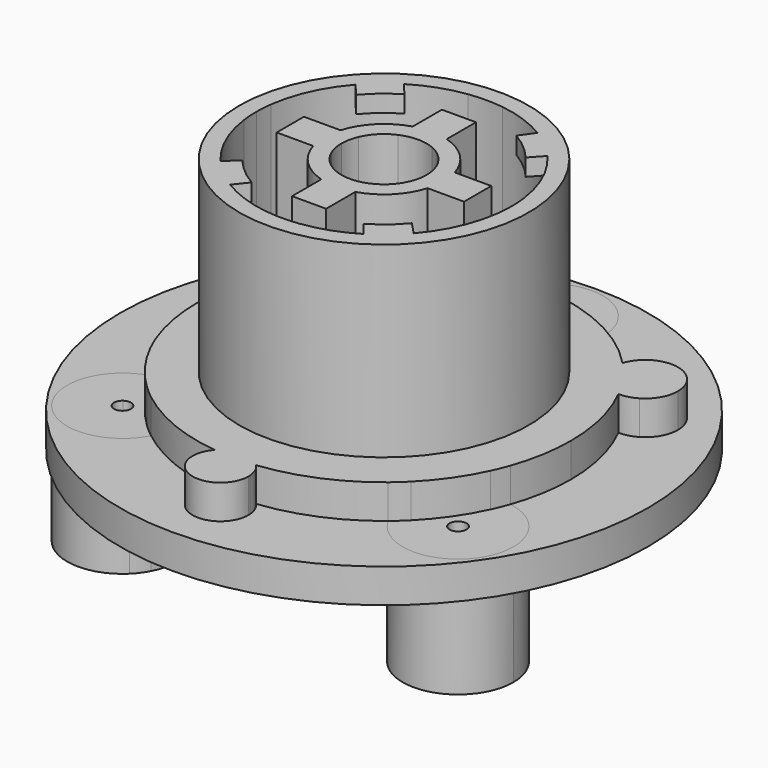
from build123d import *
from build123d import SkipClean  # not in build123d's __all__

# Parameters (mm, degrees)
F1_DEPTH  = 2
F2_DEPTH  = 15
F3_DEPTH  = 5
F4_DEPTH  = 4
F5_DEPTH  = 2
F6_DEPTH  = 1
F7_DEPTH  = 2
F8_DEPTH  = 14.99
F9_DEPTH  = 4
F12_DEPTH = 1
F14_R     = 7.5
F14_R_2   = 2.5
F15_DEPTH = 2
F16_DEPTH = 20.001


# Not quite as in the source:
# - a feature names something its author has since deleted; it is built from what else it names


with BuildPart() as f1:
    # F0 (on Top) → F1 (new body)
    with BuildSketch(Plane.XY):
        with BuildLine():
            Line((12, 0), (15.5, 0))
            ThreePointArc((15.5, 0), (0, 15.5), (-15.5, 0))
            Line((-15.5, 0), (-12, 0))
            ThreePointArc((-12, 0), (-11.6801289605, 2.7521968435), (-10.7375687557, 5.3576690095))
            ThreePointArc((-10.7375687557, 5.3576690095), (-11.2889375611, 7.9513228909), (-8.6611158458, 8.3057252727))
            ThreePointArc((-8.6611158458, 8.3057252727), (-6.1593840275, 10.2986401239), (-3.2200634035, 11.5598958333))
            ThreePointArc((-3.2200634035, 11.5598958333), (-0.2205605797, 15.2425072137), (3.25, 12))
            ThreePointArc((3.25, 12), (3.2425072137, 11.7794394203), (3.2200634035, 11.5598958333))
            ThreePointArc((3.2200634035, 11.5598958333), (6.111431372, 10.3271683721), (8.5835031281, 8.385909256))
            ThreePointArc((8.5835031281, 8.385909256), (10.6257203534, 8.6478632276), (11.7300664525, 6.9101374805))
            ThreePointArc((11.7300664525, 6.9101374805), (11.4776891115, 5.9587644605), (10.786927533, 5.2575844642))
            ThreePointArc((10.786927533, 5.2575844642), (11.692799716, 2.6978574466), (12, 0))
        make_face()
        with BuildLine():
            ThreePointArc((-15.5, 0), (0, -15.5), (15.5, 0))
            Line((15.5, 0), (12, 0))
            ThreePointArc((12, 0), (11.8294726454, -2.0158315735), (11.3227371779, -3.9743707428))
            ThreePointArc((11.3227371779, -3.9743707428), (12.6139140233, -5.1718208797), (13.090994712, -6.8669369503))
            ThreePointArc((13.090994712, -6.8669369503), (11.1449971369, -9.8438611475), (7.6374084499, -9.2558085638))
            ThreePointArc((7.6374084499, -9.2558085638), (4.8184795385, -10.9900980404), (1.6330075435, -11.8883676913))
            ThreePointArc((1.6330075435, -11.8883676913), (1.6358656226, -11.9441513269), (1.6368186856, -12))
            ThreePointArc((1.6368186856, -12), (-0.0558486731, -13.6358656226), (-1.6330075435, -11.8883676913))
            ThreePointArc((-1.6330075435, -11.8883676913), (-4.6750940722, -11.0518548405), (-7.3940132882, -9.4513791319))
            ThreePointArc((-7.3940132882, -9.4513791319), (-12.2749858869, -9.0491558433), (-11.2155025424, -4.2676108915))
            ThreePointArc((-11.2155025424, -4.2676108915), (-11.8022461953, -2.1695586523), (-12, 0))
            Line((-12, 0), (-15.5, 0))
        make_face()
        with BuildLine():
            Line((8.5, 0), (10.9707452996, 0))
            ThreePointArc((10.9707452996, 0), (10.6662314199, 2.5668579481), (9.7695945034, 4.9912198577))
            ThreePointArc((9.7695945034, 4.9912198577), (8.2415199443, 5.804885166), (7.9900576645, 7.5177277782))
            ThreePointArc((7.9900576645, 7.5177277782), (5.6655330905, 9.3946254438), (2.92083067, 10.5747813512))
            ThreePointArc((2.92083067, 10.5747813512), (0, 8.75), (-2.92083067, 10.5747813512))
            ThreePointArc((-2.92083067, 10.5747813512), (-5.7202127626, 9.3614324961), (-8.0771781233, 7.4240451232))
            ThreePointArc((-8.0771781233, 7.4240451232), (-8.0213473893, 7.1697823433), (-8.0026076616, 6.9101374805))
            ThreePointArc((-8.0026076616, 6.9101374805), (-8.4973152844, 5.667468241), (-9.7107279849, 5.1048030747))
            ThreePointArc((-9.7107279849, 5.1048030747), (-10.6510838844, 2.6290044725), (-10.9707452996, 0))
            Line((-10.9707452996, 0), (-8.5, 0))
            ThreePointArc((-8.5, 0), (0, 8.5), (8.5, 0))
        make_face()
        with BuildLine():
            ThreePointArc((10.3436272842, -3.6560398019), (10.8128292513, -1.8547172317), (10.9707452996, 0))
            Line((10.9707452996, 0), (8.5, 0))
            ThreePointArc((8.5, 0), (0, -8.5), (-8.5, 0))
            Line((-8.5, 0), (-10.9707452996, 0))
            ThreePointArc((-10.9707452996, 0), (-10.7877848856, -1.9952317382), (-10.2450061487, -3.9239140461))
            ThreePointArc((-10.2450061487, -3.9239140461), (-7.578380718, -4.6239491218), (-6.409005288, -7.120647221))
            ThreePointArc((-6.409005288, -7.120647221), (-6.5027661125, -7.8956661027), (-6.7786386831, -8.625967194))
            ThreePointArc((-6.7786386831, -8.625967194), (-4.1558671902, -10.1531285979), (-1.2150398702, -10.9032532091))
            ThreePointArc((-1.2150398702, -10.9032532091), (0, -10.3631813144), (1.2150398702, -10.9032532091))
            ThreePointArc((1.2150398702, -10.9032532091), (4.2876044557, -10.0982028331), (7.0007672753, -8.4466863317))
            ThreePointArc((7.0007672753, -8.4466863317), (7.1757253108, -5.0071415263), (10.3436272842, -3.6560398019))
        make_face()
        with BuildLine():
            ThreePointArc((-6.7786386831, -8.625967194), (-7.053433372, -9.0631958021), (-7.3940132882, -9.4513791319))
            ThreePointArc((-7.3940132882, -9.4513791319), (-4.6750940722, -11.0518548405), (-1.6330075435, -11.8883676913))
            ThreePointArc((-1.6330075435, -11.8883676913), (-1.5068032896, -11.3606884515), (-1.2150398702, -10.9032532091))
            ThreePointArc((-1.2150398702, -10.9032532091), (-4.1558671902, -10.1531285979), (-6.7786386831, -8.625967194))
        make_face()
        with BuildLine():
            Line((-10.9707452996, 0), (-12, 0))
            ThreePointArc((-12, 0), (-11.8022461953, -2.1695586523), (-11.2155025424, -4.2676108915))
            ThreePointArc((-11.2155025424, -4.2676108915), (-10.7439506432, -4.0570882487), (-10.2450061487, -3.9239140461))
            ThreePointArc((-10.2450061487, -3.9239140461), (-10.7877848856, -1.9952317382), (-10.9707452996, 0))
        make_face()
        with BuildLine():
            ThreePointArc((-10.7375687557, 5.3576690095), (-11.6801289605, 2.7521968435), (-12, 0))
            Line((-12, 0), (-10.9707452996, 0))
            ThreePointArc((-10.9707452996, 0), (-10.6510838844, 2.6290044725), (-9.7107279849, 5.1048030747))
            ThreePointArc((-9.7107279849, 5.1048030747), (-10.2430484347, 5.1544864526), (-10.7375687557, 5.3576690095))
        make_face()
        with BuildLine():
            ThreePointArc((-3.2200634035, 11.5598958333), (-6.1593840275, 10.2986401239), (-8.6611158458, 8.3057252727))
            ThreePointArc((-8.6611158458, 8.3057252727), (-8.3032471961, 7.9085306996), (-8.0771781233, 7.4240451232))
            ThreePointArc((-8.0771781233, 7.4240451232), (-5.7202127626, 9.3614324961), (-2.92083067, 10.5747813512))
            ThreePointArc((-2.92083067, 10.5747813512), (-3.1097037867, 11.0554141867), (-3.2200634035, 11.5598958333))
        make_face()
        with BuildLine():
            ThreePointArc((2.92083067, 10.5747813512), (5.6655330905, 9.3946254438), (7.9900576645, 7.5177277782))
            ThreePointArc((7.9900576645, 7.5177277782), (8.2261607277, 7.9932550925), (8.5835031281, 8.385909256))
            ThreePointArc((8.5835031281, 8.385909256), (6.111431372, 10.3271683721), (3.2200634035, 11.5598958333))
            ThreePointArc((3.2200634035, 11.5598958333), (3.1097037867, 11.0554141867), (2.92083067, 10.5747813512))
        make_face()
        with BuildLine():
            Line((10.9707452996, 0), (12, 0))
            ThreePointArc((12, 0), (11.692799716, 2.6978574466), (10.786927533, 5.2575844642))
            ThreePointArc((10.786927533, 5.2575844642), (10.2968595884, 5.0533681748), (9.7695945034, 4.9912198577))
            ThreePointArc((9.7695945034, 4.9912198577), (10.6662314199, 2.5668579481), (10.9707452996, 0))
        make_face()
        with BuildLine():
            ThreePointArc((11.3227371779, -3.9743707428), (11.8294726454, -2.0158315735), (12, 0))
            Line((12, 0), (10.9707452996, 0))
            ThreePointArc((10.9707452996, 0), (10.8128292513, -1.8547172317), (10.3436272842, -3.6560398019))
            ThreePointArc((10.3436272842, -3.6560398019), (10.8458676989, -3.7761878049), (11.3227371779, -3.9743707428))
        make_face()
        with BuildLine():
            ThreePointArc((7.6374084499, -9.2558085638), (7.2868443927, -8.8766175584), (7.0007672753, -8.4466863317))
            ThreePointArc((7.0007672753, -8.4466863317), (4.2876044557, -10.0982028331), (1.2150398702, -10.9032532091))
            ThreePointArc((1.2150398702, -10.9032532091), (1.5068032896, -11.3606884515), (1.6330075435, -11.8883676913))
            ThreePointArc((1.6330075435, -11.8883676913), (4.8184795385, -10.9900980404), (7.6374084499, -9.2558085638))
        make_face()
    extrude(amount=F1_DEPTH)

    # F0 (on Top) → F2 (join)
    with BuildSketch(Plane.XY):
        with BuildLine():
            Line((7.5, 0), (8.5, 0))
            ThreePointArc((8.5, 0), (0, 8.5), (-8.5, 0))
            Line((-8.5, 0), (-7.5, 0))
            ThreePointArc((-7.5, 0), (-7.4832398666, 0.5011198447), (-7.4330343737, 1))
            ThreePointArc((-7.4330343737, 1), (-5.3033008589, 5.3033008589), (-1, 7.4330343737))
            ThreePointArc((-1, 7.4330343737), (0, 7.5), (1, 7.4330343737))
            ThreePointArc((1, 7.4330343737), (5.3033008589, 5.3033008589), (7.4330343737, 1))
            ThreePointArc((7.4330343737, 1), (7.4832398666, 0.5011198447), (7.5, 0))
        make_face()
        with BuildLine():
            ThreePointArc((-8.5, 0), (0, -8.5), (8.5, 0))
            Line((8.5, 0), (7.5, 0))
            ThreePointArc((7.5, 0), (7.4832398666, -0.5011198447), (7.4330343737, -1))
            ThreePointArc((7.4330343737, -1), (5.3033008589, -5.3033008589), (1, -7.4330343737))
            ThreePointArc((1, -7.4330343737), (0, -7.5), (-1, -7.4330343737))
            ThreePointArc((-1, -7.4330343737), (-5.3033008589, -5.3033008589), (-7.4330343737, -1))
            ThreePointArc((-7.4330343737, -1), (-7.4832398666, -0.5011198447), (-7.5, 0))
            Line((-7.5, 0), (-8.5, 0))
        make_face()
    extrude(amount=F2_DEPTH)

    # F11 (on offset) → F12 (join)
    with BuildSketch(Plane.XY.offset(15)):
        with BuildLine():
            ThreePointArc((3.9228129696, -6.3923030596), (4.8521590221, -5.718964314), (5.6678938929, -4.9117185199))
            Line((5.6678938929, -4.9117185199), (4.9799266597, -4.1773592692))
            ThreePointArc((4.9799266597, -4.1773592692), (4.1945547803, -4.9654516607), (3.2862850661, -5.6080594205))
            Line((3.2862850661, -5.6080594205), (3.9228129696, -6.3923030596))
        make_face()
        with BuildLine():
            ThreePointArc((-5.7358275815, -4.832212946), (-4.890446416, -5.686258335), (-3.9195165937, -6.3943248018))
            Line((-3.9195165937, -6.3943248018), (-3.2862850661, -5.6080594205))
            ThreePointArc((-3.2862850661, -5.6080594205), (-4.1945547803, -4.9654516607), (-4.9799266597, -4.1773592692))
            Line((-4.9799266597, -4.1773592692), (-5.7358275815, -4.832212946))
        make_face()
        with BuildLine():
            Line((4.9799266597, 4.1773592692), (5.6618978404, 4.9186291632))
            ThreePointArc((5.6618978404, 4.9186291632), (4.8270188563, 5.7401993834), (3.8744034722, 6.421759707))
            Line((3.8744034722, 6.421759707), (3.2862850661, 5.6080594205))
            ThreePointArc((3.2862850661, 5.6080594205), (4.1945547803, 4.9654516607), (4.9799266597, 4.1773592692))
        make_face()
        with BuildLine():
            Line((-3.2862850661, 5.6080594205), (-3.9398925434, 6.3817902462))
            ThreePointArc((-3.9398925434, 6.3817902462), (-4.8398709003, 5.7293673009), (-5.633534137, 4.9510900949))
            Line((-5.633534137, 4.9510900949), (-4.9799266597, 4.1773592692))
            ThreePointArc((-4.9799266597, 4.1773592692), (-4.1945547803, 4.9654516607), (-3.2862850661, 5.6080594205))
        make_face()
    extrude(amount=-F12_DEPTH)


with BuildPart() as f3:
    # F0 (on Top) → F3 (new body)
    with BuildSketch(Plane.XY):
        with BuildLine():
            ThreePointArc((3.25, 12), (-0.2205605797, 15.2425072137), (-3.2200634035, 11.5598958333))
            ThreePointArc((-3.2200634035, 11.5598958333), (-2.7324804918, 11.6847571803), (-2.2400905501, 11.7890624872))
            ThreePointArc((-2.2400905501, 11.7890624872), (-0.1055850757, 14.2475213234), (2.2500000683, 12))
            ThreePointArc((2.2500000683, 12), (2.2475213234, 11.8944149243), (2.2400905501, 11.7890624872))
            ThreePointArc((2.2400905501, 11.7890624872), (2.7324804918, 11.6847571803), (3.2200634035, 11.5598958333))
            ThreePointArc((3.2200634035, 11.5598958333), (3.2425072137, 11.7794394203), (3.25, 12))
        make_face()
        with BuildLine():
            ThreePointArc((1.9057701678, 10.803948005), (2.4160190916, 10.7014066448), (2.92083067, 10.5747813512))
            ThreePointArc((2.92083067, 10.5747813512), (3.1097037867, 11.0554141867), (3.2200634035, 11.5598958333))
            ThreePointArc((3.2200634035, 11.5598958333), (2.7324804918, 11.6847571803), (2.2400905501, 11.7890624872))
            ThreePointArc((2.2400905501, 11.7890624872), (2.1306461248, 11.2769181248), (1.9057701678, 10.803948005))
        make_face()
        with BuildLine():
            ThreePointArc((-2.92083067, 10.5747813512), (0, 8.75), (2.92083067, 10.5747813512))
            ThreePointArc((2.92083067, 10.5747813512), (2.4160190916, 10.7014066448), (1.9057701678, 10.803948005))
            ThreePointArc((1.9057701678, 10.803948005), (0, 9.7499999317), (-1.9057701678, 10.803948005))
            ThreePointArc((-1.9057701678, 10.803948005), (-2.4160190916, 10.7014066448), (-2.92083067, 10.5747813512))
        make_face()
        with BuildLine():
            ThreePointArc((-2.2400905501, 11.7890624872), (-2.7324804918, 11.6847571803), (-3.2200634035, 11.5598958333))
            ThreePointArc((-3.2200634035, 11.5598958333), (-3.1097037867, 11.0554141867), (-2.92083067, 10.5747813512))
            ThreePointArc((-2.92083067, 10.5747813512), (-2.4160190916, 10.7014066448), (-1.9057701678, 10.803948005))
            ThreePointArc((-1.9057701678, 10.803948005), (-2.1306461248, 11.2769181248), (-2.2400905501, 11.7890624872))
        make_face()
    extrude(amount=-F3_DEPTH)


with BuildPart() as f3b:
    # F0 (on Top) → F3, piece 2 (new body)
    with BuildSketch(Plane.XY):
        with BuildLine():
            ThreePointArc((7.7695659726, -7.7453919865), (7.3934862888, -8.1051596483), (7.0007672753, -8.4466863317))
            ThreePointArc((7.0007672753, -8.4466863317), (7.2868443927, -8.8766175584), (7.6374084499, -9.2558085638))
            ThreePointArc((7.6374084499, -9.2558085638), (8.0188218667, -8.9274014063), (8.3861284242, -8.5832889997))
            ThreePointArc((8.3861284242, -8.5832889997), (8.0287565914, -8.2004635781), (7.7695659726, -7.7453919865))
        make_face()
        with BuildLine():
            ThreePointArc((13.090994712, -6.8669369503), (12.6139140233, -5.1718208797), (11.3227371779, -3.9743707428))
            ThreePointArc((11.3227371779, -3.9743707428), (11.1461170716, -4.4456804007), (10.9498885107, -4.9091691357))
            ThreePointArc((10.9498885107, -4.9091691357), (11.784896894, -5.7339124231), (12.0909947725, -6.8669369503))
            ThreePointArc((12.0909947725, -6.8669369503), (10.7867883039, -8.9084987921), (8.3861284242, -8.5832889997))
            ThreePointArc((8.3861284242, -8.5832889997), (8.0188218667, -8.9274014063), (7.6374084499, -9.2558085638))
            ThreePointArc((7.6374084499, -9.2558085638), (11.1449971369, -9.8438611475), (13.090994712, -6.8669369503))
        make_face()
        with BuildLine():
            ThreePointArc((9.950699894, -4.619612976), (10.1585947463, -4.1424878043), (10.3436272842, -3.6560398019))
            ThreePointArc((10.3436272842, -3.6560398019), (7.1757253108, -5.0071415263), (7.0007672753, -8.4466863317))
            ThreePointArc((7.0007672753, -8.4466863317), (7.3934862888, -8.1051596483), (7.7695659726, -7.7453919865))
            ThreePointArc((7.7695659726, -7.7453919865), (7.9958081538, -5.5793862374), (9.950699894, -4.619612976))
        make_face()
        with BuildLine():
            ThreePointArc((10.9498885107, -4.9091691357), (11.1461170716, -4.4456804007), (11.3227371779, -3.9743707428))
            ThreePointArc((11.3227371779, -3.9743707428), (10.8458676989, -3.7761878049), (10.3436272842, -3.6560398019))
            ThreePointArc((10.3436272842, -3.6560398019), (10.1585947463, -4.1424878043), (9.950699894, -4.619612976))
            ThreePointArc((9.950699894, -4.619612976), (10.467258683, -4.7058507162), (10.9498885107, -4.9091691357))
        make_face()
    extrude(amount=-F3_DEPTH)


with BuildPart() as f3c:
    # F0 (on Top) → F3, piece 3 (new body)
    with BuildSketch(Plane.XY):
        with BuildLine():
            ThreePointArc((-10.818459234, -5.1923924931), (-11.0266800599, -4.7341659092), (-11.2155025424, -4.2676108915))
            ThreePointArc((-11.2155025424, -4.2676108915), (-12.2749858869, -9.0491558433), (-7.3940132882, -9.4513791319))
            ThreePointArc((-7.3940132882, -9.4513791319), (-7.7838418619, -9.1330063982), (-8.1599769543, -8.7985667074))
            ThreePointArc((-8.1599769543, -8.7985667074), (-11.4700687346, -8.4557685417), (-10.818459234, -5.1923924931))
        make_face()
        with BuildLine():
            ThreePointArc((-10.2450061487, -3.9239140461), (-10.7439506432, -4.0570882487), (-11.2155025424, -4.2676108915))
            ThreePointArc((-11.2155025424, -4.2676108915), (-11.0266800599, -4.7341659092), (-10.818459234, -5.1923924931))
            ThreePointArc((-10.818459234, -5.1923924931), (-10.3412825445, -4.9765862391), (-9.8271422706, -4.8769383041))
            ThreePointArc((-9.8271422706, -4.8769383041), (-10.0473802232, -4.4053834201), (-10.2450061487, -3.9239140461))
        make_face()
        with BuildLine():
            ThreePointArc((-6.409005288, -7.120647221), (-7.578380718, -4.6239491218), (-10.2450061487, -3.9239140461))
            ThreePointArc((-10.2450061487, -3.9239140461), (-10.0473802232, -4.4053834201), (-9.8271422706, -4.8769383041))
            ThreePointArc((-9.8271422706, -4.8769383041), (-8.1286145623, -5.4712825024), (-7.4090053439, -7.120647221))
            ThreePointArc((-7.4090053439, -7.120647221), (-7.448455587, -7.5401347268), (-7.565422919, -7.9449121131))
            ThreePointArc((-7.565422919, -7.9449121131), (-7.1801103625, -8.2947735117), (-6.7786386831, -8.625967194))
            ThreePointArc((-6.7786386831, -8.625967194), (-6.5027661125, -7.8956661027), (-6.409005288, -7.120647221))
        make_face()
        with BuildLine():
            ThreePointArc((-8.1599769543, -8.7985667074), (-7.7838418619, -9.1330063982), (-7.3940132882, -9.4513791319))
            ThreePointArc((-7.3940132882, -9.4513791319), (-7.053433372, -9.0631958021), (-6.7786386831, -8.625967194))
            ThreePointArc((-6.7786386831, -8.625967194), (-7.1801103625, -8.2947735117), (-7.565422919, -7.9449121131))
            ThreePointArc((-7.565422919, -7.9449121131), (-7.8126861236, -8.4065730708), (-8.1599769543, -8.7985667074))
        make_face()
    extrude(amount=-F3_DEPTH)


with BuildPart() as f4:
    # F0 (on Top) → F4 (new body)
    with BuildSketch(Plane.XY):
        with BuildLine():
            ThreePointArc((10.3436272842, -3.6560398019), (10.8128292513, -1.8547172317), (10.9707452996, 0))
            Line((10.9707452996, 0), (8.5, 0))
            ThreePointArc((8.5, 0), (0, -8.5), (-8.5, 0))
            Line((-8.5, 0), (-10.9707452996, 0))
            ThreePointArc((-10.9707452996, 0), (-10.7877848856, -1.9952317382), (-10.2450061487, -3.9239140461))
            ThreePointArc((-10.2450061487, -3.9239140461), (-7.578380718, -4.6239491218), (-6.409005288, -7.120647221))
            ThreePointArc((-6.409005288, -7.120647221), (-6.5027661125, -7.8956661027), (-6.7786386831, -8.625967194))
            ThreePointArc((-6.7786386831, -8.625967194), (-4.1558671902, -10.1531285979), (-1.2150398702, -10.9032532091))
            ThreePointArc((-1.2150398702, -10.9032532091), (0, -10.3631813144), (1.2150398702, -10.9032532091))
            ThreePointArc((1.2150398702, -10.9032532091), (4.2876044557, -10.0982028331), (7.0007672753, -8.4466863317))
            ThreePointArc((7.0007672753, -8.4466863317), (7.1757253108, -5.0071415263), (10.3436272842, -3.6560398019))
        make_face()
        with BuildLine():
            Line((8.5, 0), (10.9707452996, 0))
            ThreePointArc((10.9707452996, 0), (10.6662314199, 2.5668579481), (9.7695945034, 4.9912198577))
            ThreePointArc((9.7695945034, 4.9912198577), (8.2415199443, 5.804885166), (7.9900576645, 7.5177277782))
            ThreePointArc((7.9900576645, 7.5177277782), (5.6655330905, 9.3946254438), (2.92083067, 10.5747813512))
            ThreePointArc((2.92083067, 10.5747813512), (0, 8.75), (-2.92083067, 10.5747813512))
            ThreePointArc((-2.92083067, 10.5747813512), (-5.7202127626, 9.3614324961), (-8.0771781233, 7.4240451232))
            ThreePointArc((-8.0771781233, 7.4240451232), (-8.0213473893, 7.1697823433), (-8.0026076616, 6.9101374805))
            ThreePointArc((-8.0026076616, 6.9101374805), (-8.4973152844, 5.667468241), (-9.7107279849, 5.1048030747))
            ThreePointArc((-9.7107279849, 5.1048030747), (-10.6510838844, 2.6290044725), (-10.9707452996, 0))
            Line((-10.9707452996, 0), (-8.5, 0))
            ThreePointArc((-8.5, 0), (0, 8.5), (8.5, 0))
        make_face()
        with BuildLine():
            ThreePointArc((-6.409005288, -7.120647221), (-7.578380718, -4.6239491218), (-10.2450061487, -3.9239140461))
            ThreePointArc((-10.2450061487, -3.9239140461), (-10.0473802232, -4.4053834201), (-9.8271422706, -4.8769383041))
            ThreePointArc((-9.8271422706, -4.8769383041), (-8.1286145623, -5.4712825024), (-7.4090053439, -7.120647221))
            ThreePointArc((-7.4090053439, -7.120647221), (-7.448455587, -7.5401347268), (-7.565422919, -7.9449121131))
            ThreePointArc((-7.565422919, -7.9449121131), (-7.1801103625, -8.2947735117), (-6.7786386831, -8.625967194))
            ThreePointArc((-6.7786386831, -8.625967194), (-6.5027661125, -7.8956661027), (-6.409005288, -7.120647221))
        make_face()
        with BuildLine():
            ThreePointArc((-7.4090053439, -7.120647221), (-8.1286145623, -5.4712825024), (-9.8271422706, -4.8769383041))
            ThreePointArc((-9.8271422706, -4.8769383041), (-8.8305405719, -6.5099005858), (-7.565422919, -7.9449121131))
            ThreePointArc((-7.565422919, -7.9449121131), (-7.448455587, -7.5401347268), (-7.4090053439, -7.120647221))
        make_face()
        with BuildLine():
            ThreePointArc((-8.0771781233, 7.4240451232), (-8.9692319542, 6.3174465237), (-9.7107279849, 5.1048030747))
            ThreePointArc((-9.7107279849, 5.1048030747), (-8.4973152844, 5.667468241), (-8.0026076616, 6.9101374805))
            ThreePointArc((-8.0026076616, 6.9101374805), (-8.0213473893, 7.1697823433), (-8.0771781233, 7.4240451232))
        make_face()
        with BuildLine():
            ThreePointArc((-8.6611158458, 8.3057252727), (-11.2889375611, 7.9513228909), (-10.7375687557, 5.3576690095))
            ThreePointArc((-10.7375687557, 5.3576690095), (-10.5507798679, 5.7167336984), (-10.351988183, 6.0692949063))
            ThreePointArc((-10.351988183, 6.0692949063), (-10.6282674714, 7.4859822706), (-9.2012987677, 7.7029929889))
            ThreePointArc((-9.2012987677, 7.7029929889), (-8.9362903661, 8.0089146888), (-8.6611158458, 8.3057252727))
        make_face()
        with BuildLine():
            ThreePointArc((-10.351988183, 6.0692949063), (-10.5507798679, 5.7167336984), (-10.7375687557, 5.3576690095))
            ThreePointArc((-10.7375687557, 5.3576690095), (-10.2430484347, 5.1544864526), (-9.7107279849, 5.1048030747))
            ThreePointArc((-9.7107279849, 5.1048030747), (-8.9692319542, 6.3174465237), (-8.0771781233, 7.4240451232))
            ThreePointArc((-8.0771781233, 7.4240451232), (-8.3032471961, 7.9085306996), (-8.6611158458, 8.3057252727))
            ThreePointArc((-8.6611158458, 8.3057252727), (-8.9362903661, 8.0089146888), (-9.2012987677, 7.7029929889))
            ThreePointArc((-9.2012987677, 7.7029929889), (-8.9136550177, 7.3520596075), (-8.8107084352, 6.9101374805))
            ThreePointArc((-8.8107084352, 6.9101374805), (-9.3317928621, 6.0322765155), (-10.351988183, 6.0692949063))
        make_face()
        with BuildLine():
            ThreePointArc((-9.2012987677, 7.7029929889), (-9.8107084352, 6.9101374805), (-10.351988183, 6.0692949063))
            ThreePointArc((-10.351988183, 6.0692949063), (-9.3317928621, 6.0322765155), (-8.8107084352, 6.9101374805))
            ThreePointArc((-8.8107084352, 6.9101374805), (-8.9136550177, 7.3520596075), (-9.2012987677, 7.7029929889))
        make_face()
        with BuildLine():
            ThreePointArc((-9.2012987677, 7.7029929889), (-10.6282674714, 7.4859822706), (-10.351988183, 6.0692949063))
            ThreePointArc((-10.351988183, 6.0692949063), (-9.8107084352, 6.9101374805), (-9.2012987677, 7.7029929889))
        make_face()
        with BuildLine():
            ThreePointArc((10.351988183, 6.0692949063), (10.5772471783, 5.667613442), (10.786927533, 5.2575844642))
            ThreePointArc((10.786927533, 5.2575844642), (11.4776891115, 5.9587644605), (11.7300664525, 6.9101374805))
            ThreePointArc((11.7300664525, 6.9101374805), (10.6257203534, 8.6478632276), (8.5835031281, 8.385909256))
            ThreePointArc((8.5835031281, 8.385909256), (8.8989543361, 8.0503796013), (9.2012987677, 7.7029929889))
            ThreePointArc((9.2012987677, 7.7029929889), (10.2526305621, 7.807190898), (10.8107084352, 6.9101374805))
            ThreePointArc((10.8107084352, 6.9101374805), (10.6885694002, 6.4312219075), (10.351988183, 6.0692949063))
        make_face()
        with BuildLine():
            ThreePointArc((9.2012987677, 7.7029929889), (9.8107084352, 6.9101374805), (10.351988183, 6.0692949063))
            ThreePointArc((10.351988183, 6.0692949063), (10.6885694002, 6.4312219075), (10.8107084352, 6.9101374805))
            ThreePointArc((10.8107084352, 6.9101374805), (10.2526305621, 7.807190898), (9.2012987677, 7.7029929889))
        make_face()
        with BuildLine():
            ThreePointArc((9.2012987677, 7.7029929889), (8.9931493989, 6.3342926905), (10.351988183, 6.0692949063))
            ThreePointArc((10.351988183, 6.0692949063), (9.8107084352, 6.9101374805), (9.2012987677, 7.7029929889))
        make_face()
        with BuildLine():
            ThreePointArc((9.7695945034, 4.9912198577), (10.2968595884, 5.0533681748), (10.786927533, 5.2575844642))
            ThreePointArc((10.786927533, 5.2575844642), (10.5772471783, 5.667613442), (10.351988183, 6.0692949063))
            ThreePointArc((10.351988183, 6.0692949063), (8.9931493989, 6.3342926905), (9.2012987677, 7.7029929889))
            ThreePointArc((9.2012987677, 7.7029929889), (8.8989543361, 8.0503796013), (8.5835031281, 8.385909256))
            ThreePointArc((8.5835031281, 8.385909256), (8.2261607277, 7.9932550925), (7.9900576645, 7.5177277782))
            ThreePointArc((7.9900576645, 7.5177277782), (8.9692319542, 6.3174465237), (9.7695945034, 4.9912198577))
        make_face()
        with BuildLine():
            ThreePointArc((7.9900576645, 7.5177277782), (8.2415199443, 5.804885166), (9.7695945034, 4.9912198577))
            ThreePointArc((9.7695945034, 4.9912198577), (8.9692319542, 6.3174465237), (7.9900576645, 7.5177277782))
        make_face()
        with BuildLine():
            ThreePointArc((7.7695659726, -7.7453919865), (8.9969205399, -6.2779513558), (9.950699894, -4.619612976))
            ThreePointArc((9.950699894, -4.619612976), (7.9958081538, -5.5793862374), (7.7695659726, -7.7453919865))
        make_face()
        with BuildLine():
            ThreePointArc((9.950699894, -4.619612976), (10.1585947463, -4.1424878043), (10.3436272842, -3.6560398019))
            ThreePointArc((10.3436272842, -3.6560398019), (7.1757253108, -5.0071415263), (7.0007672753, -8.4466863317))
            ThreePointArc((7.0007672753, -8.4466863317), (7.3934862888, -8.1051596483), (7.7695659726, -7.7453919865))
            ThreePointArc((7.7695659726, -7.7453919865), (7.9958081538, -5.5793862374), (9.950699894, -4.619612976))
        make_face()
        with BuildLine():
            ThreePointArc((0.9991315674, -11.9583333333), (0, -11), (-0.9991315674, -11.9583333333))
            ThreePointArc((-0.9991315674, -11.9583333333), (0, -12), (0.9991315674, -11.9583333333))
        make_face()
        with BuildLine():
            ThreePointArc((0.9991315674, -11.9583333333), (0, -12), (-0.9991315674, -11.9583333333))
            ThreePointArc((-0.9991315674, -11.9583333333), (-0.0208378579, -12.9997828683), (1, -12))
            ThreePointArc((1, -12), (0.9997828683, -11.9791621421), (0.9991315674, -11.9583333333))
        make_face()
        with BuildLine():
            ThreePointArc((-1.2150398702, -10.9032532091), (0, -10.9707452996), (1.2150398702, -10.9032532091))
            ThreePointArc((1.2150398702, -10.9032532091), (0, -10.3631813144), (-1.2150398702, -10.9032532091))
        make_face()
        with BuildLine():
            ThreePointArc((-0.9991315674, -11.9583333333), (-1.3165344175, -11.9275620781), (-1.6330075435, -11.8883676913))
            ThreePointArc((-1.6330075435, -11.8883676913), (-0.0558486731, -13.6358656226), (1.6368186856, -12))
            ThreePointArc((1.6368186856, -12), (1.6358656226, -11.9441513269), (1.6330075435, -11.8883676913))
            ThreePointArc((1.6330075435, -11.8883676913), (1.3165344175, -11.9275620781), (0.9991315674, -11.9583333333))
            ThreePointArc((0.9991315674, -11.9583333333), (0.9997828683, -11.9791621421), (1, -12))
            ThreePointArc((1, -12), (-0.0208378579, -12.9997828683), (-0.9991315674, -11.9583333333))
        make_face()
        with BuildLine():
            ThreePointArc((-1.2150398702, -10.9032532091), (-1.5068032896, -11.3606884515), (-1.6330075435, -11.8883676913))
            ThreePointArc((-1.6330075435, -11.8883676913), (-1.3165344175, -11.9275620781), (-0.9991315674, -11.9583333333))
            ThreePointArc((-0.9991315674, -11.9583333333), (0, -11), (0.9991315674, -11.9583333333))
            ThreePointArc((0.9991315674, -11.9583333333), (1.3165344175, -11.9275620781), (1.6330075435, -11.8883676913))
            ThreePointArc((1.6330075435, -11.8883676913), (1.5068032896, -11.3606884515), (1.2150398702, -10.9032532091))
            ThreePointArc((1.2150398702, -10.9032532091), (0, -10.9707452996), (-1.2150398702, -10.9032532091))
        make_face()
        with BuildLine():
            ThreePointArc((-1.9057701678, 10.803948005), (0, 9.7499999317), (1.9057701678, 10.803948005))
            ThreePointArc((1.9057701678, 10.803948005), (0, 10.9707452996), (-1.9057701678, 10.803948005))
        make_face()
        with BuildLine():
            ThreePointArc((-2.92083067, 10.5747813512), (0, 8.75), (2.92083067, 10.5747813512))
            ThreePointArc((2.92083067, 10.5747813512), (2.4160190916, 10.7014066448), (1.9057701678, 10.803948005))
            ThreePointArc((1.9057701678, 10.803948005), (0, 9.7499999317), (-1.9057701678, 10.803948005))
            ThreePointArc((-1.9057701678, 10.803948005), (-2.4160190916, 10.7014066448), (-2.92083067, 10.5747813512))
        make_face()
    extrude(amount=F4_DEPTH)

    # F0 (on Top) → F6 (join)
    with BuildSketch(Plane.XY):
        with BuildLine():
            ThreePointArc((-8.0771781233, 7.4240451232), (-8.9692319542, 6.3174465237), (-9.7107279849, 5.1048030747))
            ThreePointArc((-9.7107279849, 5.1048030747), (-8.4973152844, 5.667468241), (-8.0026076616, 6.9101374805))
            ThreePointArc((-8.0026076616, 6.9101374805), (-8.0213473893, 7.1697823433), (-8.0771781233, 7.4240451232))
        make_face()
        with BuildLine():
            ThreePointArc((-10.351988183, 6.0692949063), (-10.5507798679, 5.7167336984), (-10.7375687557, 5.3576690095))
            ThreePointArc((-10.7375687557, 5.3576690095), (-10.2430484347, 5.1544864526), (-9.7107279849, 5.1048030747))
            ThreePointArc((-9.7107279849, 5.1048030747), (-8.9692319542, 6.3174465237), (-8.0771781233, 7.4240451232))
            ThreePointArc((-8.0771781233, 7.4240451232), (-8.3032471961, 7.9085306996), (-8.6611158458, 8.3057252727))
            ThreePointArc((-8.6611158458, 8.3057252727), (-8.9362903661, 8.0089146888), (-9.2012987677, 7.7029929889))
            ThreePointArc((-9.2012987677, 7.7029929889), (-8.9136550177, 7.3520596075), (-8.8107084352, 6.9101374805))
            ThreePointArc((-8.8107084352, 6.9101374805), (-9.3317928621, 6.0322765155), (-10.351988183, 6.0692949063))
        make_face()
        with BuildLine():
            ThreePointArc((-8.6611158458, 8.3057252727), (-11.2889375611, 7.9513228909), (-10.7375687557, 5.3576690095))
            ThreePointArc((-10.7375687557, 5.3576690095), (-10.5507798679, 5.7167336984), (-10.351988183, 6.0692949063))
            ThreePointArc((-10.351988183, 6.0692949063), (-10.6282674714, 7.4859822706), (-9.2012987677, 7.7029929889))
            ThreePointArc((-9.2012987677, 7.7029929889), (-8.9362903661, 8.0089146888), (-8.6611158458, 8.3057252727))
        make_face()
        with BuildLine():
            ThreePointArc((7.9900576645, 7.5177277782), (8.2415199443, 5.804885166), (9.7695945034, 4.9912198577))
            ThreePointArc((9.7695945034, 4.9912198577), (8.9692319542, 6.3174465237), (7.9900576645, 7.5177277782))
        make_face()
        with BuildLine():
            ThreePointArc((9.7695945034, 4.9912198577), (10.2968595884, 5.0533681748), (10.786927533, 5.2575844642))
            ThreePointArc((10.786927533, 5.2575844642), (10.5772471783, 5.667613442), (10.351988183, 6.0692949063))
            ThreePointArc((10.351988183, 6.0692949063), (8.9931493989, 6.3342926905), (9.2012987677, 7.7029929889))
            ThreePointArc((9.2012987677, 7.7029929889), (8.8989543361, 8.0503796013), (8.5835031281, 8.385909256))
            ThreePointArc((8.5835031281, 8.385909256), (8.2261607277, 7.9932550925), (7.9900576645, 7.5177277782))
            ThreePointArc((7.9900576645, 7.5177277782), (8.9692319542, 6.3174465237), (9.7695945034, 4.9912198577))
        make_face()
        with BuildLine():
            ThreePointArc((10.351988183, 6.0692949063), (10.5772471783, 5.667613442), (10.786927533, 5.2575844642))
            ThreePointArc((10.786927533, 5.2575844642), (11.4776891115, 5.9587644605), (11.7300664525, 6.9101374805))
            ThreePointArc((11.7300664525, 6.9101374805), (10.6257203534, 8.6478632276), (8.5835031281, 8.385909256))
            ThreePointArc((8.5835031281, 8.385909256), (8.8989543361, 8.0503796013), (9.2012987677, 7.7029929889))
            ThreePointArc((9.2012987677, 7.7029929889), (10.2526305621, 7.807190898), (10.8107084352, 6.9101374805))
            ThreePointArc((10.8107084352, 6.9101374805), (10.6885694002, 6.4312219075), (10.351988183, 6.0692949063))
        make_face()
        with BuildLine():
            ThreePointArc((-1.2150398702, -10.9032532091), (0, -10.9707452996), (1.2150398702, -10.9032532091))
            ThreePointArc((1.2150398702, -10.9032532091), (0, -10.3631813144), (-1.2150398702, -10.9032532091))
        make_face()
        with BuildLine():
            ThreePointArc((-1.2150398702, -10.9032532091), (-1.5068032896, -11.3606884515), (-1.6330075435, -11.8883676913))
            ThreePointArc((-1.6330075435, -11.8883676913), (-1.3165344175, -11.9275620781), (-0.9991315674, -11.9583333333))
            ThreePointArc((-0.9991315674, -11.9583333333), (0, -11), (0.9991315674, -11.9583333333))
            ThreePointArc((0.9991315674, -11.9583333333), (1.3165344175, -11.9275620781), (1.6330075435, -11.8883676913))
            ThreePointArc((1.6330075435, -11.8883676913), (1.5068032896, -11.3606884515), (1.2150398702, -10.9032532091))
            ThreePointArc((1.2150398702, -10.9032532091), (0, -10.9707452996), (-1.2150398702, -10.9032532091))
        make_face()
        with BuildLine():
            ThreePointArc((-0.9991315674, -11.9583333333), (-1.3165344175, -11.9275620781), (-1.6330075435, -11.8883676913))
            ThreePointArc((-1.6330075435, -11.8883676913), (-0.0558486731, -13.6358656226), (1.6368186856, -12))
            ThreePointArc((1.6368186856, -12), (1.6358656226, -11.9441513269), (1.6330075435, -11.8883676913))
            ThreePointArc((1.6330075435, -11.8883676913), (1.3165344175, -11.9275620781), (0.9991315674, -11.9583333333))
            ThreePointArc((0.9991315674, -11.9583333333), (0.9997828683, -11.9791621421), (1, -12))
            ThreePointArc((1, -12), (-0.0208378579, -12.9997828683), (-0.9991315674, -11.9583333333))
        make_face()
    extrude(amount=-F6_DEPTH)

    # F0 (on Top) → F7 (cut)
    with BuildSketch(Plane.XY):
        with BuildLine():
            ThreePointArc((9.2012987677, 7.7029929889), (9.8107084352, 6.9101374805), (10.351988183, 6.0692949063))
            ThreePointArc((10.351988183, 6.0692949063), (10.6885694002, 6.4312219075), (10.8107084352, 6.9101374805))
            ThreePointArc((10.8107084352, 6.9101374805), (10.2526305621, 7.807190898), (9.2012987677, 7.7029929889))
        make_face()
        with BuildLine():
            ThreePointArc((9.2012987677, 7.7029929889), (8.9931493989, 6.3342926905), (10.351988183, 6.0692949063))
            ThreePointArc((10.351988183, 6.0692949063), (9.8107084352, 6.9101374805), (9.2012987677, 7.7029929889))
        make_face()
        with BuildLine():
            ThreePointArc((0.9991315674, -11.9583333333), (0, -11), (-0.9991315674, -11.9583333333))
            ThreePointArc((-0.9991315674, -11.9583333333), (0, -12), (0.9991315674, -11.9583333333))
        make_face()
        with BuildLine():
            ThreePointArc((0.9991315674, -11.9583333333), (0, -12), (-0.9991315674, -11.9583333333))
            ThreePointArc((-0.9991315674, -11.9583333333), (-0.0208378579, -12.9997828683), (1, -12))
            ThreePointArc((1, -12), (0.9997828683, -11.9791621421), (0.9991315674, -11.9583333333))
        make_face()
        with BuildLine():
            ThreePointArc((-9.2012987677, 7.7029929889), (-9.8107084352, 6.9101374805), (-10.351988183, 6.0692949063))
            ThreePointArc((-10.351988183, 6.0692949063), (-9.3317928621, 6.0322765155), (-8.8107084352, 6.9101374805))
            ThreePointArc((-8.8107084352, 6.9101374805), (-8.9136550177, 7.3520596075), (-9.2012987677, 7.7029929889))
        make_face()
        with BuildLine():
            ThreePointArc((-9.2012987677, 7.7029929889), (-10.6282674714, 7.4859822706), (-10.351988183, 6.0692949063))
            ThreePointArc((-10.351988183, 6.0692949063), (-9.8107084352, 6.9101374805), (-9.2012987677, 7.7029929889))
        make_face()
    with SkipClean():  # cleaning this boolean's faces spoils the solid; the shape is the same uncleaned
        extrude(amount=F7_DEPTH, mode=Mode.SUBTRACT)


with BuildPart() as f5:
    # F0 (on Top) → F5 (new body)
    with BuildSketch(Plane.XY):
        with BuildLine():
            ThreePointArc((12.0909947725, -6.8669369503), (11.784896894, -5.7339124231), (10.9498885107, -4.9091691357))
            ThreePointArc((10.9498885107, -4.9091691357), (10.5623723011, -5.6952867683), (10.1185124555, -6.4510236155))
            ThreePointArc((10.1185124555, -6.4510236155), (10.2818795449, -6.6310968262), (10.340994712, -6.8669369503))
            ThreePointArc((10.340994712, -6.8669369503), (10.0675985492, -7.3126394306), (9.5463919082, -7.2709285195))
            ThreePointArc((9.5463919082, -7.2709285195), (8.9902388108, -7.9483083813), (8.3861284242, -8.5832889997))
            ThreePointArc((8.3861284242, -8.5832889997), (10.7867883039, -8.9084987921), (12.0909947725, -6.8669369503))
        make_face()
        with BuildLine():
            ThreePointArc((13.090994712, -6.8669369503), (12.6139140233, -5.1718208797), (11.3227371779, -3.9743707428))
            ThreePointArc((11.3227371779, -3.9743707428), (11.1461170716, -4.4456804007), (10.9498885107, -4.9091691357))
            ThreePointArc((10.9498885107, -4.9091691357), (11.784896894, -5.7339124231), (12.0909947725, -6.8669369503))
            ThreePointArc((12.0909947725, -6.8669369503), (10.7867883039, -8.9084987921), (8.3861284242, -8.5832889997))
            ThreePointArc((8.3861284242, -8.5832889997), (8.0188218667, -8.9274014063), (7.6374084499, -9.2558085638))
            ThreePointArc((7.6374084499, -9.2558085638), (11.1449971369, -9.8438611475), (13.090994712, -6.8669369503))
        make_face()
        with BuildLine():
            ThreePointArc((10.1185124555, -6.4510236155), (10.5623723011, -5.6952867683), (10.9498885107, -4.9091691357))
            ThreePointArc((10.9498885107, -4.9091691357), (10.467258683, -4.7058507162), (9.950699894, -4.619612976))
            ThreePointArc((9.950699894, -4.619612976), (8.9969205399, -6.2779513558), (7.7695659726, -7.7453919865))
            ThreePointArc((7.7695659726, -7.7453919865), (8.0287565914, -8.2004635781), (8.3861284242, -8.5832889997))
            ThreePointArc((8.3861284242, -8.5832889997), (8.9902388108, -7.9483083813), (9.5463919082, -7.2709285195))
            ThreePointArc((9.5463919082, -7.2709285195), (9.4309532656, -6.5808145774), (10.1185124555, -6.4510236155))
        make_face()
        with BuildLine():
            ThreePointArc((7.7695659726, -7.7453919865), (7.3934862888, -8.1051596483), (7.0007672753, -8.4466863317))
            ThreePointArc((7.0007672753, -8.4466863317), (7.2868443927, -8.8766175584), (7.6374084499, -9.2558085638))
            ThreePointArc((7.6374084499, -9.2558085638), (8.0188218667, -8.9274014063), (8.3861284242, -8.5832889997))
            ThreePointArc((8.3861284242, -8.5832889997), (8.0287565914, -8.2004635781), (7.7695659726, -7.7453919865))
        make_face()
        with BuildLine():
            ThreePointArc((10.9498885107, -4.9091691357), (11.1461170716, -4.4456804007), (11.3227371779, -3.9743707428))
            ThreePointArc((11.3227371779, -3.9743707428), (10.8458676989, -3.7761878049), (10.3436272842, -3.6560398019))
            ThreePointArc((10.3436272842, -3.6560398019), (10.1585947463, -4.1424878043), (9.950699894, -4.619612976))
            ThreePointArc((9.950699894, -4.619612976), (10.467258683, -4.7058507162), (10.9498885107, -4.9091691357))
        make_face()
    extrude(amount=F5_DEPTH)


with BuildPart() as f5b:
    # F0 (on Top) → F5, piece 2 (new body)
    with BuildSketch(Plane.XY):
        with BuildLine():
            ThreePointArc((-8.1599769543, -8.7985667074), (-7.7838418619, -9.1330063982), (-7.3940132882, -9.4513791319))
            ThreePointArc((-7.3940132882, -9.4513791319), (-7.053433372, -9.0631958021), (-6.7786386831, -8.625967194))
            ThreePointArc((-6.7786386831, -8.625967194), (-7.1801103625, -8.2947735117), (-7.565422919, -7.9449121131))
            ThreePointArc((-7.565422919, -7.9449121131), (-7.8126861236, -8.4065730708), (-8.1599769543, -8.7985667074))
        make_face()
        with BuildLine():
            ThreePointArc((-9.8271422706, -4.8769383041), (-10.3412825445, -4.9765862391), (-10.818459234, -5.1923924931))
            ThreePointArc((-10.818459234, -5.1923924931), (-10.4106216718, -5.9681618952), (-9.9472499754, -6.7120948985))
            ThreePointArc((-9.9472499754, -6.7120948985), (-9.4289208945, -6.6767314949), (-9.159005288, -7.120647221))
            ThreePointArc((-9.159005288, -7.120647221), (-9.2103924835, -7.3414334333), (-9.3539914943, -7.5168373087))
            ThreePointArc((-9.3539914943, -7.5168373087), (-8.780403195, -8.1795183069), (-8.1599769543, -8.7985667074))
            ThreePointArc((-8.1599769543, -8.7985667074), (-7.8126861236, -8.4065730708), (-7.565422919, -7.9449121131))
            ThreePointArc((-7.565422919, -7.9449121131), (-8.8305405719, -6.5099005858), (-9.8271422706, -4.8769383041))
        make_face()
        with BuildLine():
            ThreePointArc((-10.2450061487, -3.9239140461), (-10.7439506432, -4.0570882487), (-11.2155025424, -4.2676108915))
            ThreePointArc((-11.2155025424, -4.2676108915), (-11.0266800599, -4.7341659092), (-10.818459234, -5.1923924931))
            ThreePointArc((-10.818459234, -5.1923924931), (-10.3412825445, -4.9765862391), (-9.8271422706, -4.8769383041))
            ThreePointArc((-9.8271422706, -4.8769383041), (-10.0473802232, -4.4053834201), (-10.2450061487, -3.9239140461))
        make_face()
        with BuildLine():
            ThreePointArc((-10.818459234, -5.1923924931), (-11.0266800599, -4.7341659092), (-11.2155025424, -4.2676108915))
            ThreePointArc((-11.2155025424, -4.2676108915), (-12.2749858869, -9.0491558433), (-7.3940132882, -9.4513791319))
            ThreePointArc((-7.3940132882, -9.4513791319), (-7.7838418619, -9.1330063982), (-8.1599769543, -8.7985667074))
            ThreePointArc((-8.1599769543, -8.7985667074), (-11.4700687346, -8.4557685417), (-10.818459234, -5.1923924931))
        make_face()
        with BuildLine():
            ThreePointArc((-9.9472499754, -6.7120948985), (-10.4106216718, -5.9681618952), (-10.818459234, -5.1923924931))
            ThreePointArc((-10.818459234, -5.1923924931), (-11.4700687346, -8.4557685417), (-8.1599769543, -8.7985667074))
            ThreePointArc((-8.1599769543, -8.7985667074), (-8.780403195, -8.1795183069), (-9.3539914943, -7.5168373087))
            ThreePointArc((-9.3539914943, -7.5168373087), (-10.0614638417, -7.4173408552), (-9.9472499754, -6.7120948985))
        make_face()
    extrude(amount=F5_DEPTH)


with BuildPart() as f5c:
    # F0 (on Top) → F5, piece 3 (new body)
    with BuildSketch(Plane.XY):
        with BuildLine():
            ThreePointArc((2.2500000683, 12), (-0.1055850757, 14.2475213234), (-2.2400905501, 11.7890624872))
            ThreePointArc((-2.2400905501, 11.7890624872), (-1.3736548095, 11.9211187589), (-0.4998914813, 11.9895833333))
            ThreePointArc((-0.4998914813, 11.9895833333), (-0.005208616, 12.4999728696), (0.5, 12))
            ThreePointArc((0.5, 12), (0.4999728696, 11.994791384), (0.4998914813, 11.9895833333))
            ThreePointArc((0.4998914813, 11.9895833333), (1.3736548095, 11.9211187589), (2.2400905501, 11.7890624872))
            ThreePointArc((2.2400905501, 11.7890624872), (2.2475213234, 11.8944149243), (2.2500000683, 12))
        make_face()
        with BuildLine():
            ThreePointArc((-2.2400905501, 11.7890624872), (-2.7324804918, 11.6847571803), (-3.2200634035, 11.5598958333))
            ThreePointArc((-3.2200634035, 11.5598958333), (-3.1097037867, 11.0554141867), (-2.92083067, 10.5747813512))
            ThreePointArc((-2.92083067, 10.5747813512), (-2.4160190916, 10.7014066448), (-1.9057701678, 10.803948005))
            ThreePointArc((-1.9057701678, 10.803948005), (-2.1306461248, 11.2769181248), (-2.2400905501, 11.7890624872))
        make_face()
        with BuildLine():
            ThreePointArc((-0.4998914813, 11.9895833333), (-1.3736548095, 11.9211187589), (-2.2400905501, 11.7890624872))
            ThreePointArc((-2.2400905501, 11.7890624872), (-2.1306461248, 11.2769181248), (-1.9057701678, 10.803948005))
            ThreePointArc((-1.9057701678, 10.803948005), (0, 10.9707452996), (1.9057701678, 10.803948005))
            ThreePointArc((1.9057701678, 10.803948005), (2.1306461248, 11.2769181248), (2.2400905501, 11.7890624872))
            ThreePointArc((2.2400905501, 11.7890624872), (1.3736548095, 11.9211187589), (0.4998914813, 11.9895833333))
            ThreePointArc((0.4998914813, 11.9895833333), (0, 11.5), (-0.4998914813, 11.9895833333))
        make_face()
        with BuildLine():
            ThreePointArc((1.9057701678, 10.803948005), (2.4160190916, 10.7014066448), (2.92083067, 10.5747813512))
            ThreePointArc((2.92083067, 10.5747813512), (3.1097037867, 11.0554141867), (3.2200634035, 11.5598958333))
            ThreePointArc((3.2200634035, 11.5598958333), (2.7324804918, 11.6847571803), (2.2400905501, 11.7890624872))
            ThreePointArc((2.2400905501, 11.7890624872), (2.1306461248, 11.2769181248), (1.9057701678, 10.803948005))
        make_face()
        with BuildLine():
            ThreePointArc((3.25, 12), (-0.2205605797, 15.2425072137), (-3.2200634035, 11.5598958333))
            ThreePointArc((-3.2200634035, 11.5598958333), (-2.7324804918, 11.6847571803), (-2.2400905501, 11.7890624872))
            ThreePointArc((-2.2400905501, 11.7890624872), (-0.1055850757, 14.2475213234), (2.2500000683, 12))
            ThreePointArc((2.2500000683, 12), (2.2475213234, 11.8944149243), (2.2400905501, 11.7890624872))
            ThreePointArc((2.2400905501, 11.7890624872), (2.7324804918, 11.6847571803), (3.2200634035, 11.5598958333))
            ThreePointArc((3.2200634035, 11.5598958333), (3.2425072137, 11.7794394203), (3.25, 12))
        make_face()
    extrude(amount=F5_DEPTH)


with BuildPart() as f8:
    # F0 (on Top) → F8 (new body)
    with BuildSketch(Plane.XY):
        with BuildLine():
            ThreePointArc((1, -3.354102079), (2.4748738105, -2.4748738105), (3.354102079, -1))
            Line((3.354102079, -1), (2.2912878475, -1))
            ThreePointArc((2.2912878475, -1), (1.767766953, -1.767766953), (1, -2.2912878475))
            Line((1, -2.2912878475), (1, -3.354102079))
        make_face()
        with BuildLine():
            ThreePointArc((-1, -3.354102079), (0, -3.500000108), (1, -3.354102079))
            Line((1, -3.354102079), (1, -2.2912878475))
            ThreePointArc((1, -2.2912878475), (0, -2.5), (-1, -2.2912878475))
            Line((-1, -2.2912878475), (-1, -3.354102079))
        make_face()
        with BuildLine():
            Line((-2.2912878475, -1), (-3.354102079, -1))
            ThreePointArc((-3.354102079, -1), (-2.4748738105, -2.4748738105), (-1, -3.354102079))
            Line((-1, -3.354102079), (-1, -2.2912878475))
            ThreePointArc((-1, -2.2912878475), (-1.767766953, -1.767766953), (-2.2912878475, -1))
        make_face()
        with BuildLine():
            Line((-2.5, 0), (-3.500000108, 0))
            ThreePointArc((-3.500000108, 0), (-3.4633335383, -0.5052935372), (-3.354102079, -1))
            Line((-3.354102079, -1), (-2.2912878475, -1))
            ThreePointArc((-2.2912878475, -1), (-2.4472657823, -0.5107741092), (-2.5, 0))
        make_face()
        with BuildLine():
            Line((-3.500000108, 0), (-5.5, 0))
            Line((-5.5, 0), (-5.5, -1))
            Line((-5.5, -1), (-3.354102079, -1))
            ThreePointArc((-3.354102079, -1), (-3.4633335383, -0.5052935372), (-3.500000108, 0))
        make_face()
        with BuildLine():
            Line((-5.5, 1), (-5.5, 0))
            Line((-5.5, 0), (-3.500000108, 0))
            ThreePointArc((-3.500000108, 0), (-3.4633335383, 0.5052935372), (-3.354102079, 1))
            Line((-3.354102079, 1), (-5.5, 1))
        make_face()
        with BuildLine():
            ThreePointArc((-3.354102079, 1), (-3.4633335383, 0.5052935372), (-3.500000108, 0))
            Line((-3.500000108, 0), (-2.5, 0))
            ThreePointArc((-2.5, 0), (-2.4472657823, 0.5107741092), (-2.2912878475, 1))
            Line((-2.2912878475, 1), (-3.354102079, 1))
        make_face()
        with BuildLine():
            ThreePointArc((-1, 3.354102079), (-2.4748738105, 2.4748738105), (-3.354102079, 1))
            Line((-3.354102079, 1), (-2.2912878475, 1))
            ThreePointArc((-2.2912878475, 1), (-1.767766953, 1.767766953), (-1, 2.2912878475))
            Line((-1, 2.2912878475), (-1, 3.354102079))
        make_face()
        with BuildLine():
            Line((1, 2.2912878475), (1, 3.354102079))
            ThreePointArc((1, 3.354102079), (0, 3.500000108), (-1, 3.354102079))
            Line((-1, 3.354102079), (-1, 2.2912878475))
            ThreePointArc((-1, 2.2912878475), (0, 2.5), (1, 2.2912878475))
        make_face()
        with BuildLine():
            Line((1, 3.354102079), (1, 5.5))
            Line((1, 5.5), (-1, 5.5))
            Line((-1, 5.5), (-1, 3.354102079))
            ThreePointArc((-1, 3.354102079), (0, 3.500000108), (1, 3.354102079))
        make_face()
        with BuildLine():
            Line((2.2912878475, 1), (3.354102079, 1))
            ThreePointArc((3.354102079, 1), (2.4748738105, 2.4748738105), (1, 3.354102079))
            Line((1, 3.354102079), (1, 2.2912878475))
            ThreePointArc((1, 2.2912878475), (1.767766953, 1.767766953), (2.2912878475, 1))
        make_face()
        with BuildLine():
            Line((5.5, -1), (5.5, 0))
            Line((5.5, 0), (3.500000108, 0))
            ThreePointArc((3.500000108, 0), (3.4633335383, -0.5052935372), (3.354102079, -1))
            Line((3.354102079, -1), (5.5, -1))
        make_face()
        with BuildLine():
            ThreePointArc((3.354102079, -1), (3.4633335383, -0.5052935372), (3.500000108, 0))
            Line((3.500000108, 0), (2.5, 0))
            ThreePointArc((2.5, 0), (2.4472657823, -0.5107741092), (2.2912878475, -1))
            Line((2.2912878475, -1), (3.354102079, -1))
        make_face()
        with BuildLine():
            Line((2.5, 0), (3.500000108, 0))
            ThreePointArc((3.500000108, 0), (3.4633335383, 0.5052935372), (3.354102079, 1))
            Line((3.354102079, 1), (2.2912878475, 1))
            ThreePointArc((2.2912878475, 1), (2.4472657823, 0.5107741092), (2.5, 0))
        make_face()
        with BuildLine():
            Line((3.500000108, 0), (5.5, 0))
            Line((5.5, 0), (5.5, 1))
            Line((5.5, 1), (3.354102079, 1))
            ThreePointArc((3.354102079, 1), (3.4633335383, 0.5052935372), (3.500000108, 0))
        make_face()
        with BuildLine():
            Line((-1, -5.5), (1, -5.5))
            Line((1, -5.5), (1, -3.354102079))
            ThreePointArc((1, -3.354102079), (0, -3.500000108), (-1, -3.354102079))
            Line((-1, -3.354102079), (-1, -5.5))
        make_face()
    extrude(amount=F8_DEPTH)


with BuildPart() as f9:
    # F0 (on Top) → F9 (new body)
    with BuildSketch(Plane.XY):
        with BuildLine():
            ThreePointArc((-1, -7.4330343737), (0, -7.5), (1, -7.4330343737))
            Line((1, -7.4330343737), (1, -5.5))
            Line((1, -5.5), (-1, -5.5))
            Line((-1, -5.5), (-1, -7.4330343737))
        make_face()
        with BuildLine():
            Line((-1, -5.5), (1, -5.5))
            Line((1, -5.5), (1, -3.354102079))
            ThreePointArc((1, -3.354102079), (0, -3.500000108), (-1, -3.354102079))
            Line((-1, -3.354102079), (-1, -5.5))
        make_face()
        with BuildLine():
            Line((1, 2.2912878475), (1, 3.354102079))
            ThreePointArc((1, 3.354102079), (0, 3.500000108), (-1, 3.354102079))
            Line((-1, 3.354102079), (-1, 2.2912878475))
            ThreePointArc((-1, 2.2912878475), (0, 2.5), (1, 2.2912878475))
        make_face()
        with BuildLine():
            Line((1, 3.354102079), (1, 5.5))
            Line((1, 5.5), (-1, 5.5))
            Line((-1, 5.5), (-1, 3.354102079))
            ThreePointArc((-1, 3.354102079), (0, 3.500000108), (1, 3.354102079))
        make_face()
        with BuildLine():
            ThreePointArc((-1, -3.354102079), (0, -3.500000108), (1, -3.354102079))
            Line((1, -3.354102079), (1, -2.2912878475))
            ThreePointArc((1, -2.2912878475), (0, -2.5), (-1, -2.2912878475))
            Line((-1, -2.2912878475), (-1, -3.354102079))
        make_face()
        with BuildLine():
            ThreePointArc((1, -3.354102079), (2.4748738105, -2.4748738105), (3.354102079, -1))
            Line((3.354102079, -1), (2.2912878475, -1))
            ThreePointArc((2.2912878475, -1), (1.767766953, -1.767766953), (1, -2.2912878475))
            Line((1, -2.2912878475), (1, -3.354102079))
        make_face()
        with BuildLine():
            ThreePointArc((3.354102079, -1), (3.4633335383, -0.5052935372), (3.500000108, 0))
            Line((3.500000108, 0), (2.5, 0))
            ThreePointArc((2.5, 0), (2.4472657823, -0.5107741092), (2.2912878475, -1))
            Line((2.2912878475, -1), (3.354102079, -1))
        make_face()
        with BuildLine():
            Line((2.5, 0), (3.500000108, 0))
            ThreePointArc((3.500000108, 0), (3.4633335383, 0.5052935372), (3.354102079, 1))
            Line((3.354102079, 1), (2.2912878475, 1))
            ThreePointArc((2.2912878475, 1), (2.4472657823, 0.5107741092), (2.5, 0))
        make_face()
        with BuildLine():
            Line((2.2912878475, 1), (3.354102079, 1))
            ThreePointArc((3.354102079, 1), (2.4748738105, 2.4748738105), (1, 3.354102079))
            Line((1, 3.354102079), (1, 2.2912878475))
            ThreePointArc((1, 2.2912878475), (1.767766953, 1.767766953), (2.2912878475, 1))
        make_face()
        with BuildLine():
            ThreePointArc((-1, 3.354102079), (-2.4748738105, 2.4748738105), (-3.354102079, 1))
            Line((-3.354102079, 1), (-2.2912878475, 1))
            ThreePointArc((-2.2912878475, 1), (-1.767766953, 1.767766953), (-1, 2.2912878475))
            Line((-1, 2.2912878475), (-1, 3.354102079))
        make_face()
        with BuildLine():
            ThreePointArc((-3.354102079, 1), (-3.4633335383, 0.5052935372), (-3.500000108, 0))
            Line((-3.500000108, 0), (-2.5, 0))
            ThreePointArc((-2.5, 0), (-2.4472657823, 0.5107741092), (-2.2912878475, 1))
            Line((-2.2912878475, 1), (-3.354102079, 1))
        make_face()
        with BuildLine():
            Line((-2.5, 0), (-3.500000108, 0))
            ThreePointArc((-3.500000108, 0), (-3.4633335383, -0.5052935372), (-3.354102079, -1))
            Line((-3.354102079, -1), (-2.2912878475, -1))
            ThreePointArc((-2.2912878475, -1), (-2.4472657823, -0.5107741092), (-2.5, 0))
        make_face()
        with BuildLine():
            Line((-2.2912878475, -1), (-3.354102079, -1))
            ThreePointArc((-3.354102079, -1), (-2.4748738105, -2.4748738105), (-1, -3.354102079))
            Line((-1, -3.354102079), (-1, -2.2912878475))
            ThreePointArc((-1, -2.2912878475), (-1.767766953, -1.767766953), (-2.2912878475, -1))
        make_face()
        with BuildLine():
            Line((-5.5, 0), (-7.5, 0))
            ThreePointArc((-7.5, 0), (-7.4832398666, -0.5011198447), (-7.4330343737, -1))
            Line((-7.4330343737, -1), (-5.5, -1))
            Line((-5.5, -1), (-5.5, 0))
        make_face()
        with BuildLine():
            ThreePointArc((-7.4330343737, 1), (-7.4832398666, 0.5011198447), (-7.5, 0))
            Line((-7.5, 0), (-5.5, 0))
            Line((-5.5, 0), (-5.5, 1))
            Line((-5.5, 1), (-7.4330343737, 1))
        make_face()
        with BuildLine():
            Line((-5.5, 1), (-5.5, 0))
            Line((-5.5, 0), (-3.500000108, 0))
            ThreePointArc((-3.500000108, 0), (-3.4633335383, 0.5052935372), (-3.354102079, 1))
            Line((-3.354102079, 1), (-5.5, 1))
        make_face()
        with BuildLine():
            Line((-3.500000108, 0), (-5.5, 0))
            Line((-5.5, 0), (-5.5, -1))
            Line((-5.5, -1), (-3.354102079, -1))
            ThreePointArc((-3.354102079, -1), (-3.4633335383, -0.5052935372), (-3.500000108, 0))
        make_face()
        with BuildLine():
            Line((5.5, -1), (5.5, 0))
            Line((5.5, 0), (3.500000108, 0))
            ThreePointArc((3.500000108, 0), (3.4633335383, -0.5052935372), (3.354102079, -1))
            Line((3.354102079, -1), (5.5, -1))
        make_face()
        with BuildLine():
            Line((3.500000108, 0), (5.5, 0))
            Line((5.5, 0), (5.5, 1))
            Line((5.5, 1), (3.354102079, 1))
            ThreePointArc((3.354102079, 1), (3.4633335383, 0.5052935372), (3.500000108, 0))
        make_face()
        with BuildLine():
            Line((5.5, 0), (7.5, 0))
            ThreePointArc((7.5, 0), (7.4832398666, 0.5011198447), (7.4330343737, 1))
            Line((7.4330343737, 1), (5.5, 1))
            Line((5.5, 1), (5.5, 0))
        make_face()
        with BuildLine():
            ThreePointArc((7.4330343737, -1), (7.4832398666, -0.5011198447), (7.5, 0))
            Line((7.5, 0), (5.5, 0))
            Line((5.5, 0), (5.5, -1))
            Line((5.5, -1), (7.4330343737, -1))
        make_face()
        with BuildLine():
            Line((1, 5.5), (1, 7.4330343737))
            ThreePointArc((1, 7.4330343737), (0, 7.5), (-1, 7.4330343737))
            Line((-1, 7.4330343737), (-1, 5.5))
            Line((-1, 5.5), (1, 5.5))
        make_face()
    extrude(amount=F9_DEPTH)


with BuildPart() as f15:
    # F14 (on offset) → F15 (new body)
    with BuildSketch(Plane(origin=(0, 0, 4), x_dir=(1, 0, 0), z_dir=(0, 0, -1))):
        Circle(F14_R)
        Circle(F14_R_2, mode=Mode.SUBTRACT)
    extrude(amount=F15_DEPTH)

    # F11 (on offset) → F16 (cut, through all)
    with BuildSketch(Plane.XY.offset(15)):
        with BuildLine():
            ThreePointArc((-5.7358275815, -4.832212946), (-4.890446416, -5.686258335), (-3.9195165937, -6.3943248018))
            Line((-3.9195165937, -6.3943248018), (-3.2862850661, -5.6080594205))
            ThreePointArc((-3.2862850661, -5.6080594205), (-4.1945547803, -4.9654516607), (-4.9799266597, -4.1773592692))
            Line((-4.9799266597, -4.1773592692), (-5.7358275815, -4.832212946))
        make_face()
        with BuildLine():
            ThreePointArc((3.9228129696, -6.3923030596), (4.8521590221, -5.718964314), (5.6678938929, -4.9117185199))
            Line((5.6678938929, -4.9117185199), (4.9799266597, -4.1773592692))
            ThreePointArc((4.9799266597, -4.1773592692), (4.1945547803, -4.9654516607), (3.2862850661, -5.6080594205))
            Line((3.2862850661, -5.6080594205), (3.9228129696, -6.3923030596))
        make_face()
        with BuildLine():
            Line((4.9799266597, 4.1773592692), (5.6618978404, 4.9186291632))
            ThreePointArc((5.6618978404, 4.9186291632), (4.8270188563, 5.7401993834), (3.8744034722, 6.421759707))
            Line((3.8744034722, 6.421759707), (3.2862850661, 5.6080594205))
            ThreePointArc((3.2862850661, 5.6080594205), (4.1945547803, 4.9654516607), (4.9799266597, 4.1773592692))
        make_face()
        with BuildLine():
            Line((-3.2862850661, 5.6080594205), (-3.9398925434, 6.3817902462))
            ThreePointArc((-3.9398925434, 6.3817902462), (-4.8398709003, 5.7293673009), (-5.633534137, 4.9510900949))
            Line((-5.633534137, 4.9510900949), (-4.9799266597, 4.1773592692))
            ThreePointArc((-4.9799266597, 4.1773592692), (-4.1945547803, 4.9654516607), (-3.2862850661, 5.6080594205))
        make_face()
    extrude(amount=-F16_DEPTH, mode=Mode.SUBTRACT)


solid = Compound([f1.part, f3.part, f3b.part, f3c.part, f4.part, f5.part, f5b.part, f5c.part, f8.part, f9.part, f15.part])
